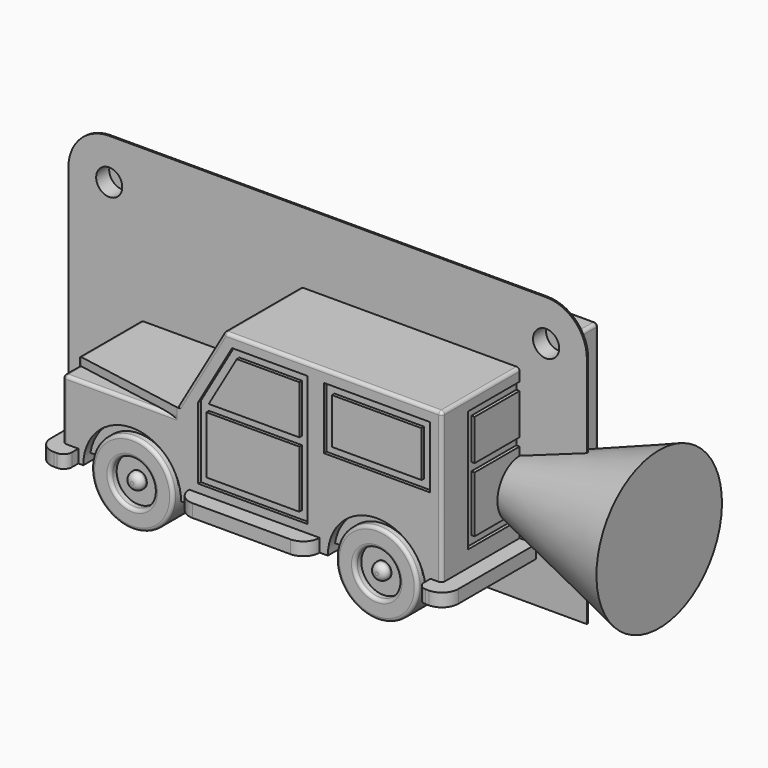
from build123d import *

# Parameters (mm, degrees)
F1_DEPTH      = 15.24
F0_R          = 6.35
F3_DEPTH      = 2.032
F4_W          = 55.9540111572
F4_H          = 9.1137220152
F5_DEPTH      = 13.97
F7_DEPTH      = 1.27
F8_R          = 1.905
F9_DEPTH      = 1.27
F10_W         = 27.94
F10_H         = 12.1246968374
F10_W_2       = 25.4
F10_H_2       = 9.5846968374
F11_DEPTH     = 0.508
F12_W         = 14.478
F12_H         = 8.9296332135
F12_W_2       = 16.51
F12_H_2       = 9.652
F12_W_3       = 13.97
F12_H_3       = 7.112
F14_DEPTH     = 0.508
F13_W         = 14.478
F13_H         = 9.0069817304
F13_W_2       = 16.51
F13_H_2       = 9.652
F13_W_3       = 13.97
F13_H_3       = 7.112
F15_DEPTH     = 0.508
F16_W         = 20.32
F16_H         = 18.923
F16_W_2       = 17.78
F16_H_2       = 8.763
F16_H_3       = 6.35
F17_DEPTH     = 0.508
F18_R         = 3.429
F18_R_2       = 1.27
F19_DEPTH     = 1.27
F20_R         = 3.429
F20_R_2       = 1.27
F21_DEPTH     = 1.27
F22_T1_DEPTH  = 33.1413576445
F22_T3_DEPTH  = 29.464
F22_T5_DEPTH  = 22.86
F22_T7_DEPTH  = 8.89
F22_T9_DEPTH  = 2.3356565316
F22_T11_DEPTH = 26.749812566
F22_S15_W     = 0.508
F22_S15_H     = 0.508
F22_T16_DEPTH = 0.508
F22_T22_DEPTH = 0.508
F22_S27_W     = 0.508
F22_S27_H     = 0.508
F22_T28_DEPTH = 0.508
F22_T34_DEPTH = 0.508
F22_S39_W     = 0.508
F22_S39_H     = 0.508
F22_T40_DEPTH = 0.508
F22_S45_W     = 0.508
F22_S45_H     = 0.508
F22_T46_DEPTH = 0.508
F22_T52_DEPTH = 20.7214029007
F22_T57_DEPTH = 20.7214029007
F22_T62_DEPTH = 18.542
F22_T67_DEPTH = 3.897093717
F22_T72_DEPTH = 3.897093717
F22_T77_DEPTH = 18.542
F22_T83_DEPTH = 3.4013130632
F22_T87_DEPTH = 3.897093717
F22_T94_DEPTH = 3.4013130632
F22_T98_DEPTH = 3.897093717
F23_R         = 0.508
F24_R         = 1.016
F26_DEPTH     = 0.127
F27_R         = 2.54
F28_DEPTH     = 3.048
F29_R         = 2.032
F30_DEPTH     = 2.54


# Not quite as in the source:
# - a fillet or chamfer that OpenCascade refuses, or shapes differently, is made with other operations: its cross-section is extruded or revolved along the edge and cut away or added


with BuildPart() as f1:
    # F0 (on Front) → F1 (new body, symmetric)
    with BuildSketch(Plane.XZ):
        with BuildLine():
            ThreePointArc((-26.67, 6.35), (-19.05, 13.97), (-11.43, 6.35))
            Line((-11.43, 6.35), (11.43, 6.35))
            ThreePointArc((11.43, 6.35), (19.05, 13.97), (26.67, 6.35))
            Line((26.67, 6.35), (29.21, 6.35))
            Line((29.21, 6.35), (29.21, 31.75))
            Line((29.21, 31.75), (-4.7326515813, 31.75))
            Line((-4.7326515813, 31.75), (-12.065, 19.05))
            Line((-12.065, 19.05), (-29.845, 19.05))
            Line((-29.845, 19.05), (-29.845, 6.35))
            Line((-29.845, 6.35), (-26.67, 6.35))
        make_face()
    extrude(amount=F1_DEPTH, both=True)

    # F2 (on face) → F3 (join)
    with BuildSketch(Plane(origin=(0, 0, 6.35), x_dir=(1, 0, 0), z_dir=(0, 0, -1))):
        with BuildLine():
            Line((7.62, 17.78), (-7.62, 17.78))
            ThreePointArc((-7.62, 17.78), (-9.4160512242, 17.0360512242), (-10.16, 15.24))
            Line((-10.16, 15.24), (-10.16, -15.24))
            ThreePointArc((-10.16, -15.24), (-9.4160512242, -17.0360512242), (-7.62, -17.78))
            Line((-7.62, -17.78), (7.62, -17.78))
            ThreePointArc((7.62, -17.78), (9.4160512242, -17.0360512242), (10.16, -15.24))
            Line((10.16, -15.24), (10.16, 15.24))
            ThreePointArc((10.16, 15.24), (9.4160512242, 17.0360512242), (7.62, 17.78))
        make_face()
        with BuildLine():
            Line((-28.702, 17.78), (-29.21, 17.78))
            ThreePointArc((-29.21, 17.78), (-31.0060512242, 17.0360512242), (-31.75, 15.24))
            Line((-31.75, 15.24), (-31.75, -15.24))
            ThreePointArc((-31.75, -15.24), (-31.0060512242, -17.0360512242), (-29.21, -17.78))
            Line((-29.21, -17.78), (-28.702, -17.78))
            ThreePointArc((-28.702, -17.78), (-27.8039743879, -17.4080256121), (-27.432, -16.51))
            Line((-27.432, -16.51), (-27.432, 16.51))
            ThreePointArc((-27.432, 16.51), (-27.8039743879, 17.4080256121), (-28.702, 17.78))
        make_face()
        with BuildLine():
            Line((29.21, 17.78), (28.702, 17.78))
            ThreePointArc((28.702, 17.78), (27.8039743879, 17.4080256121), (27.432, 16.51))
            Line((27.432, 16.51), (27.432, -16.51))
            ThreePointArc((27.432, -16.51), (27.8039743879, -17.4080256121), (28.702, -17.78))
            Line((28.702, -17.78), (29.21, -17.78))
            ThreePointArc((29.21, -17.78), (31.0060512242, -17.0360512242), (31.75, -15.24))
            Line((31.75, -15.24), (31.75, 15.24))
            ThreePointArc((31.75, 15.24), (31.0060512242, 17.0360512242), (29.21, 17.78))
        make_face()
    extrude(amount=-F3_DEPTH)



with BuildPart() as f1b:
    # F0 (on Front) → F1, piece 2 (new body, symmetric)
    with BuildSketch(Plane.XZ):
        with Locations((-19.05, 6.35)):
            Circle(F0_R)
    extrude(amount=F1_DEPTH, both=True)


with BuildPart() as f1c:
    # F0 (on Front) → F1, piece 3 (new body, symmetric)
    with BuildSketch(Plane.XZ):
        with Locations((19.05, 6.35)):
            Circle(F0_R)
    extrude(amount=F1_DEPTH, both=True)


with BuildPart() as f1_1:
    add(f1.part)

    add(f1b.part)  # F5 merges F1b

    add(f1c.part)  # F5 merges F1c
    # F4 (on Front) → F5 (join, symmetric)
    with BuildSketch(Plane.XZ):
        with Locations((0.0529857352, 12.1339668985)):
            Rectangle(F4_W, F4_H)
    extrude(amount=F5_DEPTH, both=True)

    # F6 (on face) → F7 (cut)
    with BuildSketch(Plane.XY.offset(19.05)):
        Polygon((-40.5217970916, 22.7869025582), (-34.7423643277, 11.2413688177), (-12.065, 15.24), (-14.213673774, 27.4257345109), align=None)
        Polygon((-34.7423643277, -11.2413688177), (-40.5217970916, -22.7869025582), (-14.213673774, -27.4257345109), (-12.065, -15.24), align=None)
    extrude(amount=-F7_DEPTH, mode=Mode.SUBTRACT)

    # F8 (on face) → F9 (cut)
    with BuildSketch(Plane(origin=(-29.845, 0, 0), x_dir=(0, -1, 0), z_dir=(-1, 0, 0))):
        Polygon((-6.35, 16.51), (-12.7, 16.51), (-12.7, 10.16), (-6.35, 10.16), (-6.35, 11.43), (-6.35, 12.7), (-6.35, 13.97), (-6.35, 15.24), align=None)
        with Locations((-9.525, 13.335)):
            Circle(F8_R, mode=Mode.SUBTRACT)
        Polygon((12.7, 16.51), (6.35, 16.51), (6.35, 15.24), (6.35, 13.97), (6.35, 12.7), (6.35, 11.43), (6.35, 10.16), (12.7, 10.16), align=None)
        with Locations((9.525, 13.335)):
            Circle(F8_R, mode=Mode.SUBTRACT)
        Polygon((0, 15.24), (-6.35, 15.24), (-6.35, 13.97), (0, 13.97), (6.35, 13.97), (6.35, 15.24), align=None)
        Polygon((-6.35, 12.7), (-6.35, 11.43), (0, 11.43), (6.35, 11.43), (6.35, 12.7), (0, 12.7), align=None)
    extrude(amount=-F9_DEPTH, mode=Mode.SUBTRACT)

    # F10 (on face) → F11 (cut)
    with BuildSketch(Plane(origin=(-17.297641971, 0, 9.9867982483), x_dir=(0, -1, 0), z_dir=(-0.8660254038, 0, 0.5))):
        with Locations((0, 17.7976323608)):
            Rectangle(F10_W, F10_H)
        with Locations((0, 17.7976323608)):
            Rectangle(F10_W_2, F10_H_2, mode=Mode.SUBTRACT)
    extrude(amount=-F11_DEPTH, mode=Mode.SUBTRACT)

    # F12 (on face) → F14 (cut)
    with BuildSketch(Plane.XZ.offset(15.24)):
        Polygon((-8.763, 20.8151176044), (-8.763, 9.652), (8.255, 9.652), (8.255, 26.5578628469), (8.255, 29.9606292038), (-3.4828364162, 29.9606292038), align=None)
        with Locations((-0.254, 15.3868166067)):
            Rectangle(F12_W, F12_H, mode=Mode.SUBTRACT)
        Polygon((-7.1195634468, 21.1216332135), (-2.7496015743, 28.6906292038), (6.985, 28.6906292038), (6.985, 21.1216332135), align=None, mode=Mode.SUBTRACT)
        with Locations((19.05, 25.019)):
            Rectangle(F12_W_2, F12_H_2)
        with Locations((19.05, 25.019)):
            Rectangle(F12_W_3, F12_H_3, mode=Mode.SUBTRACT)
    extrude(amount=-F14_DEPTH, mode=Mode.SUBTRACT)

    # F13 (on face) → F15 (cut)
    with BuildSketch(Plane(origin=(0, 15.24, 0), x_dir=(-1, 0, 0), z_dir=(0, 1, 0))):
        Polygon((-8.4098528528, 9.652), (8.7473845144, 9.652), (8.7473845144, 20.8924661214), (3.4672209306, 30.0379777208), (-8.255, 30.0379777208), align=None)
        with Locations((0.254, 15.4254908652)):
            Rectangle(F13_W, F13_H, mode=Mode.SUBTRACT)
        Polygon((2.7496015743, 28.7679777208), (7.1195634468, 21.1989817304), (-6.985, 21.1989817304), (-6.985, 28.7679777208), align=None, mode=Mode.SUBTRACT)
        with Locations((-19.05, 25.019)):
            Rectangle(F13_W_2, F13_H_2)
        with Locations((-19.05, 25.019)):
            Rectangle(F13_W_3, F13_H_3, mode=Mode.SUBTRACT)
    extrude(amount=-F15_DEPTH, mode=Mode.SUBTRACT)

    # F16 (on face) → F17 (cut)
    with BuildSketch(Plane.YZ.offset(29.21)):
        with Locations((0, 20.3835)):
            Rectangle(F16_W, F16_H)
        with Locations((0, 16.5735)):
            Rectangle(F16_W_2, F16_H_2, mode=Mode.SUBTRACT)
        with Locations((0, 25.4)):
            Rectangle(F16_W_2, F16_H_3, mode=Mode.SUBTRACT)
    extrude(amount=-F17_DEPTH, mode=Mode.SUBTRACT)

    # F18 (on face) → F19 (cut)
    with BuildSketch(Plane.XZ.offset(15.24)):
        with Locations((19.05, 6.35)):
            Circle(F18_R)
        with Locations((19.05, 6.35)):
            Circle(F18_R_2, mode=Mode.SUBTRACT)
        with Locations((-19.05, 6.35)):
            Circle(F18_R)
        with Locations((-19.05, 6.35)):
            Circle(F18_R_2, mode=Mode.SUBTRACT)
    extrude(amount=-F19_DEPTH, mode=Mode.SUBTRACT)

    # F20 (on face) → F21 (cut)
    with BuildSketch(Plane(origin=(0, 15.24, 0), x_dir=(-1, 0, 0), z_dir=(0, 1, 0))):
        with Locations((-19.05, 6.35)):
            Circle(F20_R)
        with Locations((-19.05, 6.35)):
            Circle(F20_R_2, mode=Mode.SUBTRACT)
        with Locations((19.05, 6.35)):
            Circle(F20_R)
        with Locations((19.05, 6.35)):
            Circle(F20_R_2, mode=Mode.SUBTRACT)
    extrude(amount=-F21_DEPTH, mode=Mode.SUBTRACT)

    # F22: fillet of radius 0.508 on 17 edges, made by hand

    # F22_s2 → F22_t1 (cut)
    with BuildSketch(Plane.YZ.offset(-4.4393576445)):
        with BuildLine():
            ThreePointArc((15.24, 31.242), (15.0912102448, 31.6012102448), (14.732, 31.75))
            Line((14.732, 31.75), (15.24, 31.75))
            Line((15.24, 31.75), (15.24, 31.242))
        make_face()
        with BuildLine():
            ThreePointArc((-15.24, 31.242), (-15.0912102448, 31.6012102448), (-14.732, 31.75))
            Line((-14.732, 31.75), (-15.24, 31.75))
            Line((-15.24, 31.75), (-15.24, 31.242))
        make_face()
    extrude(amount=F22_T1_DEPTH, mode=Mode.SUBTRACT)

    # F22_s4 → F22_t3 (cut)
    with BuildSketch(Plane.XZ.offset(-14.732)):
        with BuildLine():
            ThreePointArc((-4.4393576445, 31.75), (-4.6933576445, 31.6819409051), (-4.8792985497, 31.496))
            Line((-4.8792985497, 31.496), (-4.7326515813, 31.75))
            Line((-4.7326515813, 31.75), (-4.4393576445, 31.75))
        make_face()
        with BuildLine():
            ThreePointArc((28.702, 31.75), (29.0612102448, 31.6012102448), (29.21, 31.242))
            Line((29.21, 31.242), (29.21, 31.75))
            Line((29.21, 31.75), (28.702, 31.75))
        make_face()
    extrude(amount=F22_T3_DEPTH, mode=Mode.SUBTRACT)

    # F22_s6 → F22_t5 (cut)
    with BuildSketch(Plane.XY.offset(8.382)):
        with BuildLine():
            ThreePointArc((28.702, -15.24), (29.0612102448, -15.0912102448), (29.21, -14.732))
            Line((29.21, -14.732), (29.21, -15.24))
            Line((29.21, -15.24), (28.702, -15.24))
        make_face()
        with BuildLine():
            ThreePointArc((28.702, 15.24), (29.0612102448, 15.0912102448), (29.21, 14.732))
            Line((29.21, 14.732), (29.21, 15.24))
            Line((29.21, 15.24), (28.702, 15.24))
        make_face()
    extrude(amount=F22_T5_DEPTH, mode=Mode.SUBTRACT)

    # F22_s8 → F22_t7 (cut)
    with BuildSketch(Plane.XY.offset(8.382)):
        with BuildLine():
            ThreePointArc((-29.337, -15.24), (-29.6962102448, -15.0912102448), (-29.845, -14.732))
            Line((-29.845, -14.732), (-29.845, -15.24))
            Line((-29.845, -15.24), (-29.337, -15.24))
        make_face()
        with BuildLine():
            ThreePointArc((-29.337, 15.24), (-29.6962102448, 15.0912102448), (-29.845, 14.732))
            Line((-29.845, 14.732), (-29.845, 15.24))
            Line((-29.845, 15.24), (-29.337, 15.24))
        make_face()
    extrude(amount=F22_T7_DEPTH, mode=Mode.SUBTRACT)

    # F22_s10 → F22_t9 (cut)
    with BuildSketch(Plane.XY.offset(17.78)):
        with BuildLine():
            ThreePointArc((-29.845, -11.6786436704), (-29.7261505771, -12.0051797761), (-29.4252132743, -12.1789260089))
            Line((-29.4252132743, -12.1789260089), (-29.845, -12.104906283))
            Line((-29.845, -12.104906283), (-29.845, -11.6786436704))
        make_face()
        with BuildLine():
            ThreePointArc((-29.4252132743, 12.1789260089), (-29.7261505771, 12.0051797761), (-29.845, 11.6786436704))
            Line((-29.845, 11.6786436704), (-29.845, 12.104906283))
            Line((-29.845, 12.104906283), (-29.4252132743, 12.1789260089))
        make_face()
    extrude(amount=F22_T9_DEPTH, mode=Mode.SUBTRACT)

    # F22_s12 → F22_t11 (cut)
    with BuildSketch(Plane.XZ.offset(-13.374906283)):
        with BuildLine():
            ThreePointArc((-29.845, 18.542), (-29.6962102448, 18.9012102448), (-29.337, 19.05))
            Line((-29.337, 19.05), (-29.845, 19.05))
            Line((-29.845, 19.05), (-29.845, 18.542))
        make_face()
    extrude(amount=F22_T11_DEPTH, mode=Mode.SUBTRACT)


with BuildPart() as f22_tool14:
    # F22_s15 → F22_t16 (new body)
    with BuildSketch(Plane.XY.offset(31.242)):
        with Locations((28.956, 14.986)):
            Rectangle(F22_S15_W, F22_S15_H)
    extrude(amount=F22_T16_DEPTH)

    # F22_s17 → F22_t18 (revolve, cut)
    with BuildSketch(Plane(origin=(28.702, 14.732, 31.242), x_dir=(-0.7071067812, -0.7071067812, 0), z_dir=(-0.7071067812, 0.7071067812, 0))):
        with BuildLine():
            ThreePointArc((0, -0.508), (0.508, 0), (0, 0.508))
            Line((0, 0.508), (0, -0.508))
        make_face()
    revolve(axis=Axis((28.702, 14.732, 31.242), (0, 0, 1)), mode=Mode.SUBTRACT)


with BuildPart() as f1_2:
    add(f1_1.part)

    # F22_t13: cut F22_tool14
    add(f22_tool14.part, mode=Mode.SUBTRACT)


with BuildPart() as f22_tool20:
    # F22_s21 → F22_t22 (new body)
    with BuildSketch(Plane.XZ.offset(-14.732)):
        Polygon((-4.4393576445, 31.242), (-4.4393576445, 31.75), (-4.7326515813, 31.75), (-4.8792985497, 31.496), align=None)
    extrude(amount=-F22_T22_DEPTH)

    # F22_s23 → F22_t24 (revolve, cut)
    with BuildSketch(Plane(origin=(-4.4393576445, 14.732, 31.242), x_dir=(0.5, 0, -0.8660254038), z_dir=(0.8660254038, 0, 0.5))):
        with BuildLine():
            ThreePointArc((0, -0.508), (0.508, 0), (0, 0.508))
            Line((0, 0.508), (0, -0.508))
        make_face()
    revolve(axis=Axis((-4.4393576445, 14.732, 31.242), (0, 1, 0)), mode=Mode.SUBTRACT)


with BuildPart() as f1_3:
    add(f1_2.part)

    # F22_t19: cut F22_tool20
    add(f22_tool20.part, mode=Mode.SUBTRACT)


with BuildPart() as f22_tool26:
    # F22_s27 → F22_t28 (new body)
    with BuildSketch(Plane.XY.offset(31.242)):
        with Locations((28.956, -14.986)):
            Rectangle(F22_S27_W, F22_S27_H)
    extrude(amount=F22_T28_DEPTH)

    # F22_s29 → F22_t30 (revolve, cut)
    with BuildSketch(Plane(origin=(28.702, -14.732, 31.242), x_dir=(-0.7071067812, 0.7071067812, 0), z_dir=(0.7071067812, 0.7071067812, 0))):
        with BuildLine():
            ThreePointArc((0, -0.508), (0.508, 0), (0, 0.508))
            Line((0, 0.508), (0, -0.508))
        make_face()
    revolve(axis=Axis((28.702, -14.732, 31.242), (0, 0, 1)), mode=Mode.SUBTRACT)


with BuildPart() as f1_4:
    add(f1_3.part)

    # F22_t25: cut F22_tool26
    add(f22_tool26.part, mode=Mode.SUBTRACT)


with BuildPart() as f22_tool32:
    # F22_s33 → F22_t34 (new body)
    with BuildSketch(Plane.XZ.offset(14.732)):
        Polygon((-4.4393576445, 31.242), (-4.4393576445, 31.75), (-4.7326515813, 31.75), (-4.8792985497, 31.496), align=None)
    extrude(amount=F22_T34_DEPTH)

    # F22_s35 → F22_t36 (revolve, cut)
    with BuildSketch(Plane(origin=(-4.4393576445, -14.732, 31.242), x_dir=(0.5, 0, -0.8660254038), z_dir=(-0.8660254038, 0, -0.5))):
        with BuildLine():
            ThreePointArc((0, -0.508), (0.508, 0), (0, 0.508))
            Line((0, 0.508), (0, -0.508))
        make_face()
    revolve(axis=Axis((-4.4393576445, -14.732, 31.242), (0, -1, 0)), mode=Mode.SUBTRACT)


with BuildPart() as f1_5:
    add(f1_4.part)

    # F22_t31: cut F22_tool32
    add(f22_tool32.part, mode=Mode.SUBTRACT)


with BuildPart() as f22_tool38:
    # F22_s39 → F22_t40 (new body)
    with BuildSketch(Plane.XY.offset(17.272)):
        with Locations((-29.591, -14.986)):
            Rectangle(F22_S39_W, F22_S39_H)
    extrude(amount=F22_T40_DEPTH)

    # F22_s41 → F22_t42 (revolve, cut)
    with BuildSketch(Plane(origin=(-29.337, -14.732, 17.272), x_dir=(0.7071067812, 0.7071067812, 0), z_dir=(0.7071067812, -0.7071067812, 0))):
        with BuildLine():
            ThreePointArc((0, -0.508), (0.508, 0), (0, 0.508))
            Line((0, 0.508), (0, -0.508))
        make_face()
    revolve(axis=Axis((-29.337, -14.732, 17.272), (0, 0, 1)), mode=Mode.SUBTRACT)


with BuildPart() as f1_6:
    add(f1_5.part)

    # F22_t37: cut F22_tool38
    add(f22_tool38.part, mode=Mode.SUBTRACT)


with BuildPart() as f22_tool44:
    # F22_s45 → F22_t46 (new body)
    with BuildSketch(Plane.YZ.offset(-29.337)):
        with Locations((14.986, 17.526)):
            Rectangle(F22_S45_W, F22_S45_H)
    extrude(amount=-F22_T46_DEPTH)

    # F22_s47 → F22_t48 (revolve, cut)
    with BuildSketch(Plane(origin=(-29.337, 14.732, 17.272), x_dir=(0, -0.7071067812, -0.7071067812), z_dir=(0, 0.7071067812, -0.7071067812))):
        with BuildLine():
            ThreePointArc((0, -0.508), (0.508, 0), (0, 0.508))
            Line((0, 0.508), (0, -0.508))
        make_face()
    revolve(axis=Axis((-29.337, 14.732, 17.272), (-1, 0, 0)), mode=Mode.SUBTRACT)


with BuildPart() as f1_7:
    add(f1_6.part)

    # F22_t43: cut F22_tool44
    add(f22_tool44.part, mode=Mode.SUBTRACT)


with BuildPart() as f22_tool50:
    # F22_s51 → F22_t52 (new body)
    with BuildSketch(Plane(origin=(12.4183434214, 0, 21.5092017517), x_dir=(0, 1, 0), z_dir=(-0.5, 0, -0.8660254038))):
        with BuildLine():
            ThreePointArc((-15.24, -19.4655964967), (-15.0912102448, -19.8248067415), (-14.732, -19.9735964967))
            Line((-14.732, -19.9735964967), (-15.24, -19.9735964967))
            Line((-15.24, -19.9735964967), (-15.24, -19.4655964967))
        make_face()
    extrude(amount=F22_T52_DEPTH)

    split(bisect_by=Plane.XY.offset(19.05), keep=Keep.TOP)


with BuildPart() as f1_8:
    add(f1_7.part)

    # F22_t49: cut F22_tool50
    add(f22_tool50.part, mode=Mode.SUBTRACT)


with BuildPart() as f22_tool55:
    # F22_s56 → F22_t57 (new body)
    with BuildSketch(Plane(origin=(12.4183434214, 0, 21.5092017517), x_dir=(0, 1, 0), z_dir=(-0.5, 0, -0.8660254038))):
        with BuildLine():
            ThreePointArc((15.24, -19.4655964967), (15.0912102448, -19.8248067415), (14.732, -19.9735964967))
            Line((14.732, -19.9735964967), (15.24, -19.9735964967))
            Line((15.24, -19.9735964967), (15.24, -19.4655964967))
        make_face()
    extrude(amount=F22_T57_DEPTH)

    split(bisect_by=Plane.XY.offset(19.05), keep=Keep.TOP)


with BuildPart() as f1_9:
    add(f1_8.part)

    # F22_t54: cut F22_tool55
    add(f22_tool55.part, mode=Mode.SUBTRACT)


with BuildPart() as f22_tool60:
    # F22_s61 → F22_t62 (new body)
    with BuildSketch(Plane.YZ.offset(-10.795)):
        with BuildLine():
            ThreePointArc((-15.24, 17.272), (-15.0912102448, 17.6312102448), (-14.732, 17.78))
            Line((-14.732, 17.78), (-15.24, 17.78))
            Line((-15.24, 17.78), (-15.24, 17.272))
        make_face()
    extrude(amount=-F22_T62_DEPTH)

    split(bisect_by=Plane(origin=(-2.9699977573, -16.843694285, 0), x_dir=(0, 0, 1), z_dir=(-0.1736481777, -0.984807753, 0)), keep=Keep.TOP)


with BuildPart() as f1_10:
    add(f1_9.part)

    # F22_t59: cut F22_tool60
    add(f22_tool60.part, mode=Mode.SUBTRACT)


with BuildPart() as f22_tool65:
    # F22_s66 → F22_t67 (new body)
    with BuildSketch(Plane.XZ.offset(14.732)):
        with BuildLine():
            ThreePointArc((-29.845, 17.272), (-29.6962102448, 17.6312102448), (-29.337, 17.78))
            Line((-29.337, 17.78), (-29.845, 17.78))
            Line((-29.845, 17.78), (-29.845, 17.272))
        make_face()
    extrude(amount=-F22_T67_DEPTH)

    split(bisect_by=Plane(origin=(-2.9699977573, -16.843694285, 0), x_dir=(0, 0, 1), z_dir=(-0.1736481777, -0.984807753, 0)), keep=Keep.TOP)


with BuildPart() as f1_11:
    add(f1_10.part)

    # F22_t64: cut F22_tool65
    add(f22_tool65.part, mode=Mode.SUBTRACT)


with BuildPart() as f22_tool70:
    # F22_s71 → F22_t72 (new body)
    with BuildSketch(Plane.XZ.offset(-10.834906283)):
        with BuildLine():
            ThreePointArc((-29.337, 17.78), (-29.6962102448, 17.6312102448), (-29.845, 17.272))
            Line((-29.845, 17.272), (-29.845, 17.78))
            Line((-29.845, 17.78), (-29.337, 17.78))
        make_face()
    extrude(amount=-F22_T72_DEPTH)

    split(bisect_by=Plane(origin=(-2.9699977573, 16.843694285, 0), x_dir=(0, 0, 1), z_dir=(-0.1736481777, 0.984807753, 0)), keep=Keep.TOP)


with BuildPart() as f1_12:
    add(f1_11.part)

    # F22_t69: cut F22_tool70
    add(f22_tool70.part, mode=Mode.SUBTRACT)


with BuildPart() as f22_tool75:
    # F22_s76 → F22_t77 (new body)
    with BuildSketch(Plane.YZ.offset(-10.795)):
        with BuildLine():
            ThreePointArc((15.24, 17.272), (15.0912102448, 17.6312102448), (14.732, 17.78))
            Line((14.732, 17.78), (15.24, 17.78))
            Line((15.24, 17.78), (15.24, 17.272))
        make_face()
    extrude(amount=-F22_T77_DEPTH)

    split(bisect_by=Plane(origin=(-2.9699977573, 16.843694285, 0), x_dir=(0, 0, 1), z_dir=(-0.1736481777, 0.984807753, 0)), keep=Keep.TOP)


with BuildPart() as f1_13:
    add(f1_12.part)

    # F22_t74: cut F22_tool75
    add(f22_tool75.part, mode=Mode.SUBTRACT)


with BuildPart() as f22_tool81:
    # F22_s82 → F22_t83 (new body)
    with BuildSketch(Plane.XY.offset(20.1156565316)):
        with BuildLine():
            ThreePointArc((-29.845, -11.6786436704), (-29.7261505771, -12.0051797761), (-29.4252132743, -12.1789260089))
            Line((-29.4252132743, -12.1789260089), (-29.845, -12.104906283))
            Line((-29.845, -12.104906283), (-29.845, -11.6786436704))
        make_face()
    extrude(amount=-F22_T83_DEPTH)

    split(bisect_by=Plane.XY.offset(17.78), keep=Keep.BOTTOM)


with BuildPart() as f22_tool85:
    # F22_s86 → F22_t87 (new body)
    with BuildSketch(Plane.XZ.offset(14.732)):
        with BuildLine():
            ThreePointArc((-29.845, 17.272), (-29.6962102448, 17.6312102448), (-29.337, 17.78))
            Line((-29.337, 17.78), (-29.845, 17.78))
            Line((-29.845, 17.78), (-29.845, 17.272))
        make_face()
    extrude(amount=-F22_T87_DEPTH)

    split(bisect_by=Plane(origin=(-2.9699977573, -16.843694285, 0), x_dir=(0, 0, 1), z_dir=(0.1736481777, 0.984807753, 0)), keep=Keep.TOP)


with BuildPart() as f22_tool81_1:
    add(f22_tool81.part)

    # F22_t89: intersect F22_tool85
    add(f22_tool85.part, mode=Mode.INTERSECT)


with BuildPart() as f1_14:
    add(f1_13.part)

    # F22_t79: cut F22_tool81
    add(f22_tool81_1.part, mode=Mode.SUBTRACT)


with BuildPart() as f22_tool92:
    # F22_s93 → F22_t94 (new body)
    with BuildSketch(Plane.XY.offset(16.7143434684)):
        with BuildLine():
            ThreePointArc((-29.4252132743, 12.1789260089), (-29.7261505771, 12.0051797761), (-29.845, 11.6786436704))
            Line((-29.845, 11.6786436704), (-29.845, 12.104906283))
            Line((-29.845, 12.104906283), (-29.4252132743, 12.1789260089))
        make_face()
    extrude(amount=F22_T94_DEPTH)

    split(bisect_by=Plane.XY.offset(17.78), keep=Keep.BOTTOM)


with BuildPart() as f22_tool96:
    # F22_s97 → F22_t98 (new body)
    with BuildSketch(Plane.XZ.offset(-10.834906283)):
        with BuildLine():
            ThreePointArc((-29.337, 17.78), (-29.6962102448, 17.6312102448), (-29.845, 17.272))
            Line((-29.845, 17.272), (-29.845, 17.78))
            Line((-29.845, 17.78), (-29.337, 17.78))
        make_face()
    extrude(amount=-F22_T98_DEPTH)

    split(bisect_by=Plane(origin=(-2.9699977573, 16.843694285, 0), x_dir=(0, 0, 1), z_dir=(0.1736481777, -0.984807753, 0)), keep=Keep.TOP)


with BuildPart() as f22_tool92_1:
    add(f22_tool92.part)

    # F22_t100: intersect F22_tool96
    add(f22_tool96.part, mode=Mode.INTERSECT)


with BuildPart() as f1_15:
    add(f1_14.part)

    # F22_t90: cut F22_tool92
    add(f22_tool92_1.part, mode=Mode.SUBTRACT)

    # F23
    f23_edges = [f1_15.edges().sort_by_distance(p)[0] for p in [
        (-25.4, -15.24, 6.35),
        (12.7, -15.24, 6.35),
        (-22.479, -15.24, 6.35),
        (15.621, -15.24, 6.35),
        (22.479, 15.24, 6.35),
        (12.7, 15.24, 6.35),
        (-15.621, 15.24, 6.35),
        (-25.4, 15.24, 6.35),
    ]]
    fillet(f23_edges, radius=F23_R)

    # F24
    f24_edges = [f1_15.edges().sort_by_distance(p)[0] for p in [
        (20.32, 15.24, 6.35),
        (-17.78, 15.24, 6.35),
        (-20.32, -15.24, 6.35),
        (17.78, -15.24, 6.35),
    ]]
    fillet(f24_edges, radius=F24_R)

    # F25 (on Front) → F26 (join, symmetric)
    with BuildSketch(Plane.XZ):
        with BuildLine():
            Line((33.3370784461, 42.7603088319), (-34.714735502, 42.7603088319))
            ThreePointArc((-34.714735502, 42.7603088319), (-39.2048635625, 40.9004368925), (-41.064735502, 36.4103088319))
            Line((-41.064735502, 36.4103088319), (-41.064735502, 0))
            Line((-41.064735502, 0), (39.6870784461, 0))
            Line((39.6870784461, 0), (39.6870784461, 36.4103088319))
            ThreePointArc((39.6870784461, 36.4103088319), (37.8272065067, 40.9004368925), (33.3370784461, 42.7603088319))
        make_face()
    extrude(amount=F26_DEPTH, both=True)

    # F27 (on face) → F28 (join)
    with BuildSketch(Plane.XZ.offset(0.127)):
        with Locations((33.3370784461, 36.4103088319)):
            Circle(F27_R)
        with Locations((-34.714735502, 36.4103088319)):
            Circle(F27_R)
    extrude(amount=-F28_DEPTH)

    # F29 (on face) → F30 (cut)
    with BuildSketch(Plane.XZ.offset(0.127)):
        with Locations((-34.714735502, 36.4103088319)):
            Circle(F29_R)
        with Locations((33.3370784461, 36.4103088319)):
            Circle(F29_R)
    extrude(amount=-F30_DEPTH, mode=Mode.SUBTRACT)

    # F31 (on Front) → F32 (revolve)
    with BuildSketch(Plane.XZ):
        Polygon((50.8531149808, 27.457738925), (23.4065372497, 17.6009964198), (23.1108969884, 15.24), (50.8531149808, 15.24), align=None)
    revolve(axis=Axis((53.107372952, 0, 15.24), (1, 0, 0)))


solid = f1_15.part
